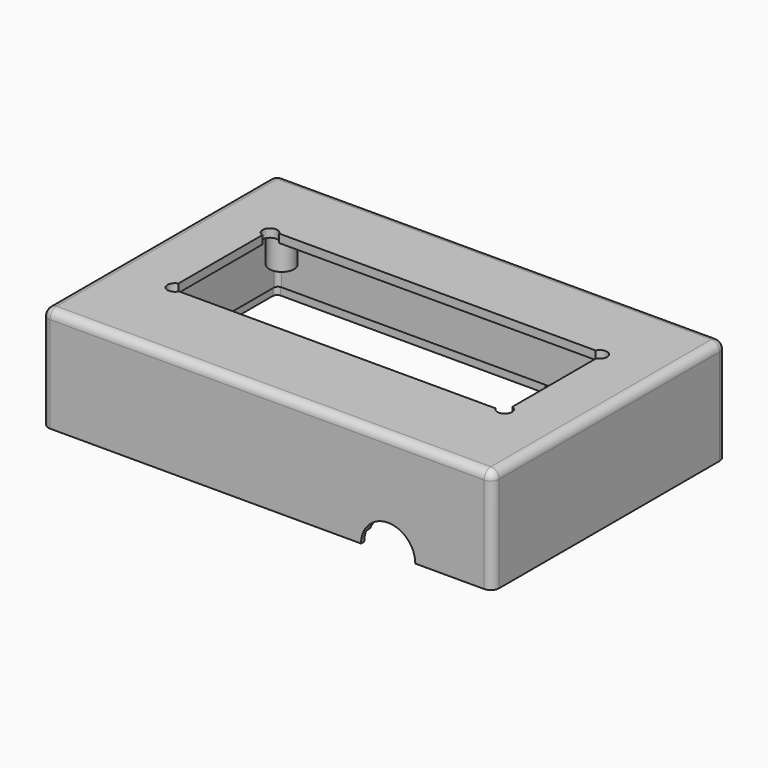
from build123d import *

# Parameters (mm, degrees)
F0_W      = 104
F0_H      = 66
F0_R      = 3
F1_DEPTH  = 2
F2_DEPTH  = 22.49
F3_DEPTH  = 23
F4_DEPTH  = 14
F6_DEPTH  = 2.5
F7_W      = 21
F7_H      = 2.4
F8_DEPTH  = 2.5
F10_D     = 2.4384
F10_DEPTH = 10
F10_TIP   = 0.7325692667
F11_R     = 2
F12_R     = 1


with BuildPart() as f1:
    # F0 (on Top) → F1 (new body)
    with BuildSketch(Plane.XY):
        with BuildLine():
            Line((48.4044117422, 34.8920698583), (-55.5955882578, 34.8920698583))
            ThreePointArc((-55.5955882578, 34.8920698583), (-57.0098018202, 34.3062834207), (-57.5955882578, 32.8920698583))
            Line((-57.5955882578, 32.8920698583), (-57.5955882578, -33.1079301417))
            ThreePointArc((-57.5955882578, -33.1079301417), (-57.0098018202, -34.5221437041), (-55.5955882578, -35.1079301417))
            Line((-55.5955882578, -35.1079301417), (48.4044117422, -35.1079301417))
            ThreePointArc((48.4044117422, -35.1079301417), (49.8186253046, -34.5221437041), (50.4044117422, -33.1079301417))
            Line((50.4044117422, -33.1079301417), (50.4044117422, 32.8920698583))
            ThreePointArc((50.4044117422, 32.8920698583), (49.8186253046, 34.3062834207), (48.4044117422, 34.8920698583))
        make_face()
        with BuildLine():
            ThreePointArc((-56.6455882578, 32.8920698583), (-56.338050378, 33.6345319786), (-55.5955882578, 33.9420698583))
            Line((-55.5955882578, 33.9420698583), (48.4044117422, 33.9420698583))
            ThreePointArc((48.4044117422, 33.9420698583), (49.1468738625, 33.6345319786), (49.4544117422, 32.8920698583))
            Line((49.4544117422, 32.8920698583), (49.4544117422, -33.1079301417))
            ThreePointArc((49.4544117422, -33.1079301417), (49.1468738625, -33.8503922619), (48.4044117422, -34.1579301417))
            Line((48.4044117422, -34.1579301417), (-55.5955882578, -34.1579301417))
            ThreePointArc((-55.5955882578, -34.1579301417), (-56.338050378, -33.8503922619), (-56.6455882578, -33.1079301417))
            Line((-56.6455882578, -33.1079301417), (-56.6455882578, 32.8920698583))
        make_face(mode=Mode.SUBTRACT)
        with BuildLine():
            Line((48.4044117422, 33.9420698583), (-55.5955882578, 33.9420698583))
            ThreePointArc((-55.5955882578, 33.9420698583), (-56.338050378, 33.6345319786), (-56.6455882578, 32.8920698583))
            Line((-56.6455882578, 32.8920698583), (-56.6455882578, -33.1079301417))
            ThreePointArc((-56.6455882578, -33.1079301417), (-56.338050378, -33.8503922619), (-55.5955882578, -34.1579301417))
            Line((-55.5955882578, -34.1579301417), (48.4044117422, -34.1579301417))
            ThreePointArc((48.4044117422, -34.1579301417), (49.1468738625, -33.8503922619), (49.4544117422, -33.1079301417))
            Line((49.4544117422, -33.1079301417), (49.4544117422, 32.8920698583))
            ThreePointArc((49.4544117422, 32.8920698583), (49.1468738625, 33.6345319786), (48.4044117422, 33.9420698583))
        make_face()
        with Locations((-3.5955882578, -0.1079301417)):
            Rectangle(F0_W, F0_H, mode=Mode.SUBTRACT)
        with Locations((-3.5955882578, -0.1079301417)):
            Rectangle(F0_W, F0_H)
        with Locations((-50.0955882578, -27.6079301417)):
            Circle(F0_R, mode=Mode.SUBTRACT)
        with Locations((42.9044117422, -27.6079301417)):
            Circle(F0_R, mode=Mode.SUBTRACT)
        with Locations((-50.0955882578, 27.3920698583)):
            Circle(F0_R, mode=Mode.SUBTRACT)
        with BuildLine():
            ThreePointArc((-43.5955882578, 13.4650188752), (-44.424068371, 16.2812101433), (-41.5144494277, 15.8920698583))
            Line((-41.5144494277, 15.8920698583), (34.3232729121, 15.8920698583))
            ThreePointArc((34.3232729121, 15.8920698583), (36.2887989476, 16.8493327192), (37.6544117422, 15.1420698583))
            ThreePointArc((37.6544117422, 15.1420698583), (37.3075332623, 14.0962448251), (36.4044117422, 13.4650188752))
            Line((36.4044117422, 13.4650188752), (36.4044117422, -11.6808791586))
            ThreePointArc((36.4044117422, -11.6808791586), (37.3075332623, -12.3121051085), (37.6544117422, -13.3579301417))
            ThreePointArc((37.6544117422, -13.3579301417), (36.2887989476, -15.0651930026), (34.3232729121, -14.1079301417))
            Line((34.3232729121, -14.1079301417), (-41.5144494277, -14.1079301417))
            ThreePointArc((-41.5144494277, -14.1079301417), (-44.424068371, -14.4970704267), (-43.5955882578, -11.6808791586))
            Line((-43.5955882578, -11.6808791586), (-43.5955882578, 13.4650188752))
        make_face(mode=Mode.SUBTRACT)
        with Locations((42.9044117422, 27.3920698583)):
            Circle(F0_R, mode=Mode.SUBTRACT)
        with Locations((-50.0955882578, 27.3920698583)):
            Circle(F0_R)
        with Locations((42.9044117422, 27.3920698583)):
            Circle(F0_R)
        with Locations((42.9044117422, -27.6079301417)):
            Circle(F0_R)
        with Locations((-50.0955882578, -27.6079301417)):
            Circle(F0_R)
    extrude(amount=-F1_DEPTH)

    # F0 (on Top) → F2 (join)
    with BuildSketch(Plane.XY):
        with BuildLine():
            Line((48.4044117422, 33.9420698583), (-55.5955882578, 33.9420698583))
            ThreePointArc((-55.5955882578, 33.9420698583), (-56.338050378, 33.6345319786), (-56.6455882578, 32.8920698583))
            Line((-56.6455882578, 32.8920698583), (-56.6455882578, -33.1079301417))
            ThreePointArc((-56.6455882578, -33.1079301417), (-56.338050378, -33.8503922619), (-55.5955882578, -34.1579301417))
            Line((-55.5955882578, -34.1579301417), (48.4044117422, -34.1579301417))
            ThreePointArc((48.4044117422, -34.1579301417), (49.1468738625, -33.8503922619), (49.4544117422, -33.1079301417))
            Line((49.4544117422, -33.1079301417), (49.4544117422, 32.8920698583))
            ThreePointArc((49.4544117422, 32.8920698583), (49.1468738625, 33.6345319786), (48.4044117422, 33.9420698583))
        make_face()
        with Locations((-3.5955882578, -0.1079301417)):
            Rectangle(F0_W, F0_H, mode=Mode.SUBTRACT)
    extrude(amount=-F2_DEPTH)

    # F3 (add): a face of the model
    f3_faces = [f1.faces().sort_by_distance(p)[0] for p in [
        (-3.5955882578, 34.763368654, -2),
    ]]
    extrude(f3_faces, amount=F3_DEPTH)

    # F0 (on Top) → F4 (join)
    with BuildSketch(Plane.XY):
        with Locations((-50.0955882578, 27.3920698583)):
            Circle(F0_R)
        with Locations((42.9044117422, 27.3920698583)):
            Circle(F0_R)
        with Locations((-50.0955882578, -27.6079301417)):
            Circle(F0_R)
        with Locations((42.9044117422, -27.6079301417)):
            Circle(F0_R)
    extrude(amount=-F4_DEPTH)

    # F5 (on face) → F6 (cut)
    with BuildSketch(Plane.XZ.offset(35.1079301417)):
        with BuildLine():
            Line((18.9044117422, -25), (31.9044117422, -25))
            ThreePointArc((31.9044117422, -25), (25.4044117422, -18.5), (18.9044117422, -25))
        make_face()
    extrude(amount=-F6_DEPTH, mode=Mode.SUBTRACT)

    # F7 (on face) → F8 (cut)
    with BuildSketch(Plane(origin=(0, 34.8920698583, 0), x_dir=(-1, 0, 0), z_dir=(0, 1, 0))):
        with Locations((-18.3044117422, -23.8)):
            Rectangle(F7_W, F7_H)
    extrude(amount=-F8_DEPTH, mode=Mode.SUBTRACT)

    # F10
    with Locations(Plane(origin=(0, 0, -14), x_dir=(1, 0, 0), z_dir=(0, 0, -1))):
        with Locations((-50.0955882578, -27.3920698583), (42.9044117422, -27.3920698583), (42.9044117422, 27.6079301417), (-50.0955882578, 27.6079301417)):
            Hole(F10_D / 2, depth=F10_DEPTH)
            with Locations((0, 0, -(F10_DEPTH + F10_TIP / 2))):  # 118° drill point
                Cone(0, F10_D / 2, F10_TIP, mode=Mode.SUBTRACT)

    # F11
    f11_edges = [f1.edges().sort_by_distance(p)[0] for p in [
        (-57.595588, -0.10793, 0),
        (-3.595588, 34.89207, 0),
        (50.404412, -0.10793, 0),
        (-3.595588, -35.10793, 0),
        (-57.009802, 34.306283, 0),
        (-57.009802, -34.522144, 0),
        (49.818625, -34.522144, 0),
        (49.818625, 34.306283, 0),
    ]]
    fillet(f11_edges, radius=F11_R)

    # F12
    f12_edges = [f1.edges().sort_by_distance(p)[0] for p in [
        (48.404412, -33.10793, -12.245),
        (48.404412, -0.10793, -2),
        (-3.595588, -33.10793, -2),
        (-55.595588, -33.10793, -12.245),
        (-55.595588, -0.10793, -2),
        (-55.595588, 32.89207, -12.245),
        (-3.595588, 32.89207, -2),
        (48.404412, 32.89207, -12.245),
    ]]
    fillet(f12_edges, radius=F12_R)


solid = f1.part
